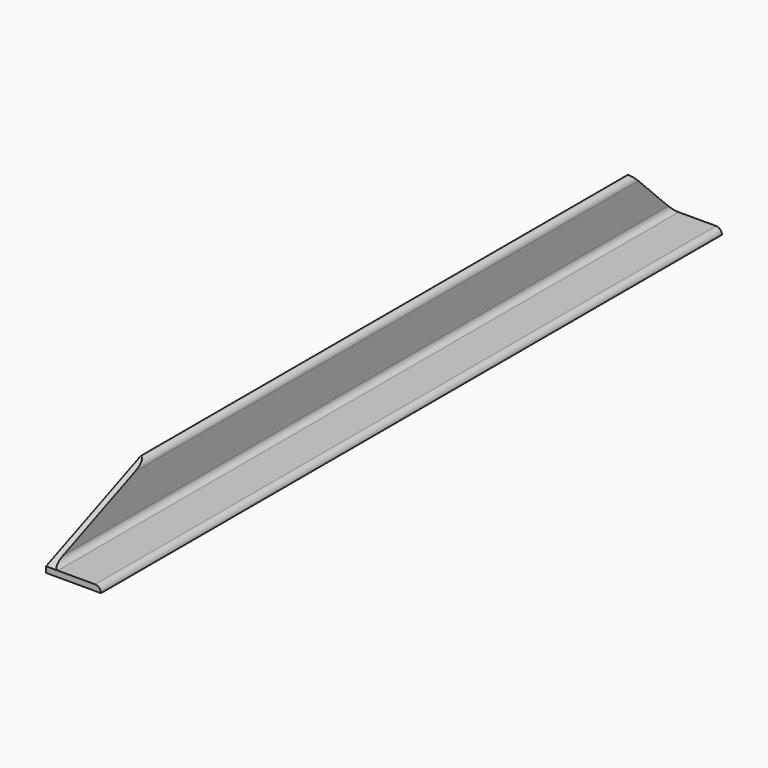
from build123d import *

# Parameters (mm, degrees)
F1_DEPTH = 628.65
F2_R     = 4.76249
F4_DEPTH = 25.4


# Not quite as in the source:
# - a fillet or chamfer is up to 0.001 mm smaller than in the source, because OpenCascade refuses the exact size


with BuildPart() as f1:
    # F0 (on Front) → F1 (new body)
    with BuildSketch(Plane.XZ):
        Polygon((0, 44.45), (0, 0), (44.45, 0), (44.45, 4.7625), (4.7625, 4.7625), (4.7625, 44.45), align=None)
    extrude(amount=F1_DEPTH)

    # F2 (radius 4.7625 in the source; OpenCascade refuses exactly that, so slightly less here)
    f2_edges = [f1.edges().sort_by_distance(p)[0] for p in [
        (4.7625, -314.325, 4.7625),
        (4.7625, -314.325, 44.45),
        (44.45, -314.325, 4.7625),
    ]]
    fillet(f2_edges, radius=F2_R)

    # F3 (on face) → F4 (cut)
    with BuildSketch(Plane(origin=(0, 0, 0), x_dir=(0, -1, 0), z_dir=(-1, 0, 0))):
        Polygon((0, 44.45), (0, 4.7625), (39.6875, 44.45), align=None)
        Polygon((628.65, 44.45), (532.8358992433, 44.45), (628.65, 4.7625), align=None)
    extrude(amount=-F4_DEPTH, mode=Mode.SUBTRACT)


solid = f1.part
